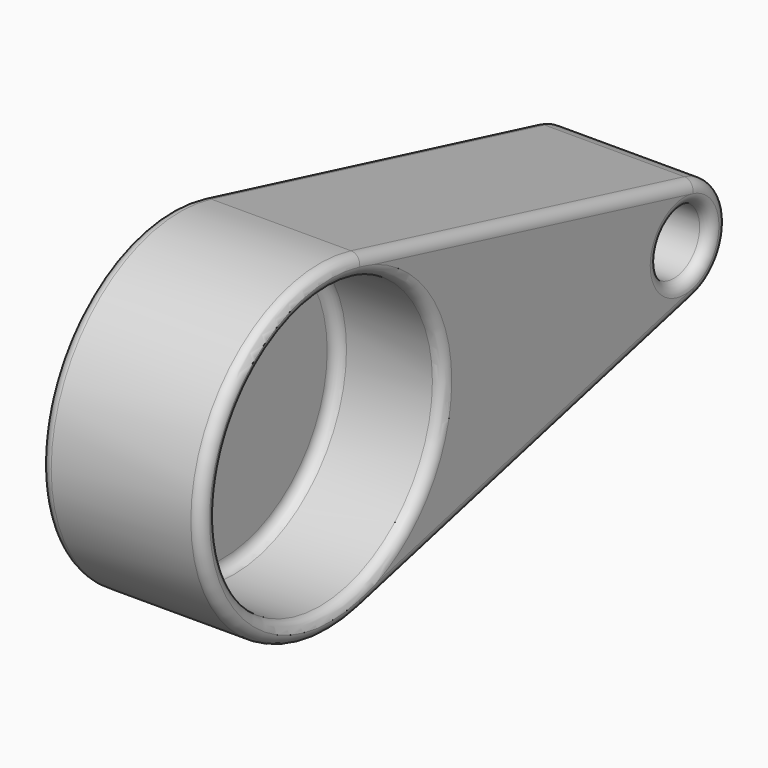
from build123d import *

# Parameters (mm, degrees)
F1_DEPTH     = 76.2
F2_R         = 66.675
F2_R_2       = 15.24
F3_DEPTH     = 50.8
F4_T5_DEPTH  = 203.2
F4_T7_DEPTH  = 203.2
F4_T10_ANGLE = 208.0724869359
F4_T12_ANGLE = 151.9275130641
F4_T18_ANGLE = 208.0724869359
F4_T20_ANGLE = 151.9275130641
F5_T         = -2.54


# Not quite as in the source:
# - a fillet or chamfer that OpenCascade refuses, or shapes differently, is made with other operations: its cross-section is extruded or revolved along the edge and cut away or added
# - a shell that OpenCascade refuses in one call is made with other operations: the cavity is built on its own and cut out


with BuildPart() as f1:
    # F0 (on Right) → F1 (new body)
    with BuildSketch(Plane.YZ):
        with BuildLine():
            ThreePointArc((18.4812146278, -73.9248585111), (60.0612543768, -46.8944103565), (76.2, 0))
            ThreePointArc((76.2, 0), (60.0612543768, 46.8944103565), (18.4812146278, 73.9248585111))
            ThreePointArc((18.4812146278, 73.9248585111), (-76.2, 0), (18.4812146278, -73.9248585111))
        make_face()
        with BuildLine():
            ThreePointArc((18.4812146278, 73.9248585111), (60.0612543768, 46.8944103565), (76.2, 0))
            ThreePointArc((76.2, 0), (60.0612543768, -46.8944103565), (18.4812146278, -73.9248585111))
            Line((18.4812146278, -73.9248585111), (215.6141706573, -24.6416195037))
            ThreePointArc((215.6141706573, -24.6416195037), (184.0537657814, 0), (215.6141706573, 24.6416195037))
            Line((215.6141706573, 24.6416195037), (18.4812146278, 73.9248585111))
        make_face()
        with BuildLine():
            ThreePointArc((234.8537657814, 0), (229.474183907, 15.6314701188), (215.6141706573, 24.6416195037))
            ThreePointArc((215.6141706573, 24.6416195037), (184.0537657814, 0), (215.6141706573, -24.6416195037))
            ThreePointArc((215.6141706573, -24.6416195037), (229.474183907, -15.6314701188), (234.8537657814, 0))
        make_face()
    extrude(amount=F1_DEPTH)

    # F2 (on face) → F3 (cut)
    with BuildSketch(Plane.YZ.offset(76.2)):
        Circle(F2_R)
        with Locations((209.4537657814, 0)):
            Circle(F2_R_2)
    extrude(amount=-F3_DEPTH, mode=Mode.SUBTRACT)

    # F4: fillet of radius 5.08 on 12 edges, made by hand

    # F4_s1 → F4_t2 (revolve)
    with BuildSketch(Plane.XY):
        with BuildLine():
            ThreePointArc((30.48, 66.675), (26.8878975516, 65.1871024484), (25.4, 61.595))
            Line((25.4, 61.595), (25.4, 66.675))
            Line((25.4, 66.675), (30.48, 66.675))
        make_face()
    revolve(axis=Axis((25.4, 0, 0), (1, 0, 0)))

    # F4_s3 → F4_t4 (revolve)
    with BuildSketch(Plane.XY):
        with BuildLine():
            ThreePointArc((30.48, 224.6937657814), (26.8878975516, 223.2058682298), (25.4, 219.6137657814))
            Line((25.4, 219.6137657814), (25.4, 224.6937657814))
            Line((25.4, 224.6937657814), (30.48, 224.6937657814))
        make_face()
    revolve(axis=Axis((25.4, 209.4537657814, 0), (1, 0, 0)))

    # F4_s6 → F4_t5 (cut)
    with BuildSketch(Plane(origin=(0, 197.1329560295, -49.2832390074), x_dir=(1, 0, 0), z_dir=(0, -0.9701425001, 0.242535625))):
        with BuildLine():
            ThreePointArc((71.12, 76.2), (74.7121024484, 74.7121024484), (76.2, 71.12))
            Line((76.2, 71.12), (76.2, 76.2))
            Line((76.2, 76.2), (71.12, 76.2))
        make_face()
        with BuildLine():
            ThreePointArc((5.08, 76.2), (1.4878975516, 74.7121024484), (0, 71.12))
            Line((0, 71.12), (0, 76.2))
            Line((0, 76.2), (5.08, 76.2))
        make_face()
    extrude(amount=F4_T5_DEPTH, mode=Mode.SUBTRACT)

    # F4_s8 → F4_t7 (cut)
    with BuildSketch(Plane(origin=(0, 0, 0), x_dir=(1, 0, 0), z_dir=(0, 0.9701425001, 0.242535625))):
        with BuildLine():
            ThreePointArc((71.12, 76.2), (74.7121024484, 74.7121024484), (76.2, 71.12))
            Line((76.2, 71.12), (76.2, 76.2))
            Line((76.2, 76.2), (71.12, 76.2))
        make_face()
        with BuildLine():
            ThreePointArc((5.08, 76.2), (1.4878975516, 74.7121024484), (0, 71.12))
            Line((0, 71.12), (0, 76.2))
            Line((0, 76.2), (5.08, 76.2))
        make_face()
    extrude(amount=F4_T7_DEPTH, mode=Mode.SUBTRACT)

    # F4_s9 → F4_t10 (revolve, cut)
    with BuildSketch(Plane(origin=(0, 0, 0), x_dir=(1, 0, 0), z_dir=(0, 0.9701425001, -0.242535625))):
        with BuildLine():
            ThreePointArc((71.12, -76.2), (74.7121024484, -74.7121024484), (76.2, -71.12))
            Line((76.2, -71.12), (76.2, -76.2))
            Line((76.2, -76.2), (71.12, -76.2))
        make_face()
    revolve(axis=Axis((76.2, 0, 0), (1, 0, 0)), revolution_arc=F4_T10_ANGLE, mode=Mode.SUBTRACT)

    # F4_s11 → F4_t12 (revolve, cut)
    with BuildSketch(Plane(origin=(0, 197.1329560295, 49.2832390074), x_dir=(1, 0, 0), z_dir=(0, -0.9701425001, -0.242535625))):
        with BuildLine():
            ThreePointArc((76.2, -71.12), (74.7121024484, -74.7121024484), (71.12, -76.2))
            Line((71.12, -76.2), (76.2, -76.2))
            Line((76.2, -76.2), (76.2, -71.12))
        make_face()
    revolve(axis=Axis((76.2, 209.4537657814, 0), (1, 0, 0)), revolution_arc=F4_T12_ANGLE, mode=Mode.SUBTRACT)

    # F4_s13 → F4_t14 (revolve, cut)
    with BuildSketch(Plane.XY):
        with BuildLine():
            ThreePointArc((76.2, 71.755), (74.7121024484, 68.1628975516), (71.12, 66.675))
            Line((71.12, 66.675), (76.2, 66.675))
            Line((76.2, 66.675), (76.2, 71.755))
        make_face()
    revolve(axis=Axis((76.2, 0, 0), (1, 0, 0)), mode=Mode.SUBTRACT)

    # F4_s15 → F4_t16 (revolve, cut)
    with BuildSketch(Plane.XY):
        with BuildLine():
            ThreePointArc((76.2, 229.7737657814), (74.7121024484, 226.1816633329), (71.12, 224.6937657814))
            Line((71.12, 224.6937657814), (76.2, 224.6937657814))
            Line((76.2, 224.6937657814), (76.2, 229.7737657814))
        make_face()
    revolve(axis=Axis((76.2, 209.4537657814, 0), (1, 0, 0)), mode=Mode.SUBTRACT)

    # F4_s17 → F4_t18 (revolve, cut)
    with BuildSketch(Plane(origin=(0, 0, 0), x_dir=(1, 0, 0), z_dir=(0, 0.9701425001, -0.242535625))):
        with BuildLine():
            ThreePointArc((5.08, -76.2), (1.4878975516, -74.7121024484), (0, -71.12))
            Line((0, -71.12), (0, -76.2))
            Line((0, -76.2), (5.08, -76.2))
        make_face()
    revolve(axis=Axis((0, 0, 0), (1, 0, 0)), revolution_arc=F4_T18_ANGLE, mode=Mode.SUBTRACT)

    # F4_s19 → F4_t20 (revolve, cut)
    with BuildSketch(Plane(origin=(0, 197.1329560295, 49.2832390074), x_dir=(1, 0, 0), z_dir=(0, -0.9701425001, -0.242535625))):
        with BuildLine():
            ThreePointArc((0, -71.12), (1.4878975516, -74.7121024484), (5.08, -76.2))
            Line((5.08, -76.2), (0, -76.2))
            Line((0, -76.2), (0, -71.12))
        make_face()
    revolve(axis=Axis((0, 209.4537657814, 0), (1, 0, 0)), revolution_arc=F4_T20_ANGLE, mode=Mode.SUBTRACT)

    # F5: a shell. OpenCascade refuses it in one call, so the cavity is built on its own and cut out:
    # the body offset inwards by the wall thickness, plus a prism from it out through each open face.
    f5_core = offset(f1.part, amount=F5_T, mode=Mode.PRIVATE)
    f5_exits = [f5_core.faces().sort_by_distance(p)[0] for p in [
        (2.54, 56.038662, 0),
    ]]
    add(f5_core, mode=Mode.SUBTRACT)
    extrude(f5_exits, amount=-F5_T, mode=Mode.SUBTRACT)


solid = f1.part
